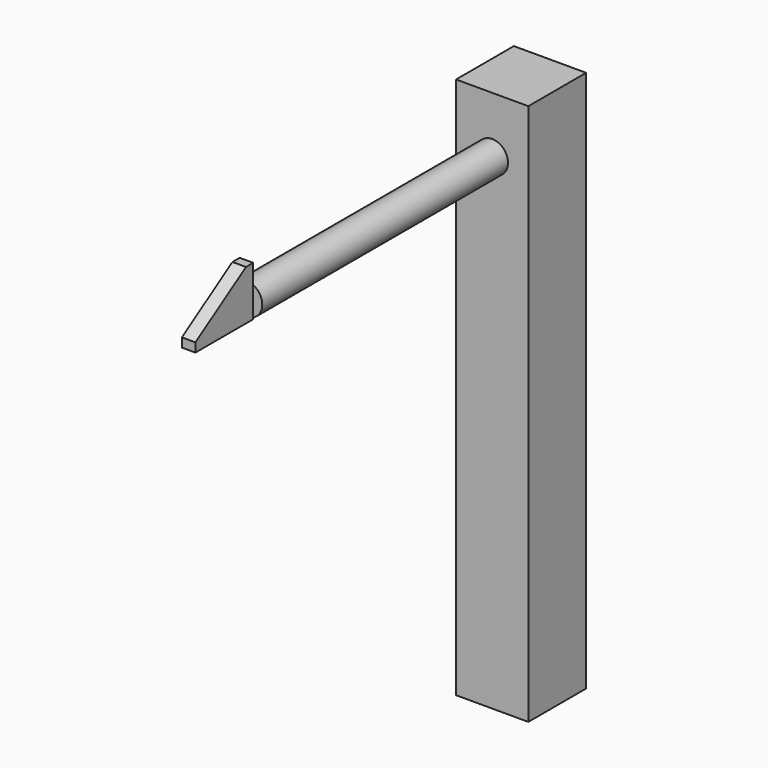
from build123d import *

# Parameters (mm, degrees)
F0_W          = 50.8
F0_H          = 50.8
F1_DEPTH      = 381
F2_R          = 11.1125
F3_DEPTH      = 215.9
F5_DEPTH      = 4.7625
F5_DEPTH_BACK = 4.7625


# Not quite as in the source:
# - the program builds the solid bodies; features that only make, move or delete a surface that nothing else refers to are left out


with BuildPart() as f1:
    # F0 (on Top) → F1 (new body)
    with BuildSketch(Plane.XY):
        Rectangle(F0_W, F0_H)
    extrude(amount=F1_DEPTH)

    # F2 (on face) → F3 (join)
    with BuildSketch(Plane.XZ.offset(25.4)):
        with Locations((0, 341.3125)):
            Circle(F2_R)
    extrude(amount=F3_DEPTH)

    # F4 (on Right) → F5 (join, two sides)
    with BuildSketch(Plane.YZ) as f5_sk:
        Polygon((-292.1, 330.2), (-241.3, 330.2), (-241.3, 365.125), (-247.65, 365.125), (-292.1, 336.55), align=None)
    extrude(amount=F5_DEPTH)
    extrude(f5_sk.sketch, amount=-F5_DEPTH_BACK)


solid = f1.part
